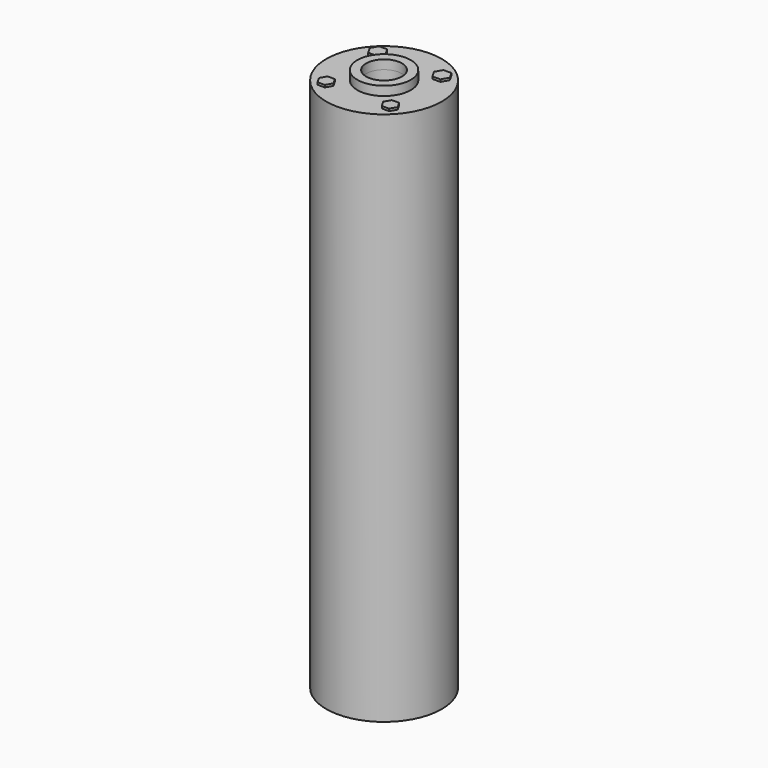
from build123d import *

# Parameters (mm, degrees)
F0_R      = 12.954
F0_R_2    = 5.9944
F0_R_3    = 4.0132
F1_DEPTH  = 119.888
F2_R      = 5.9944
F2_R_2    = 4.0132
F3_DEPTH  = 2.032
F5_R      = 5.9944
F5_R_2    = 4.0132
F6_DEPTH  = 2.032
F7_R      = 4.0132
F8_DEPTH  = 50.8
F10_DEPTH = 0.508


# Not quite as in the source:
# - the program builds the solid bodies; features that only make, move or delete a surface that nothing else refers to are left out


with BuildPart() as f1:
    # F0 (on Top) → F1 (new body)
    with BuildSketch(Plane.XY):
        Circle(F0_R)
        Circle(F0_R_2, mode=Mode.SUBTRACT)
        Circle(F0_R_2)
        Circle(F0_R_3, mode=Mode.SUBTRACT)
        Circle(F0_R_3)
    extrude(amount=F1_DEPTH)

    # F2 (on face) → F3 (join)
    with BuildSketch(Plane.XY.offset(119.888)):
        Circle(F2_R)
        Circle(F2_R_2, mode=Mode.SUBTRACT)
    extrude(amount=F3_DEPTH)

    # F5 (on face) + F0 (on Top) → F6 (join)
    with BuildSketch(Plane.XY):
        Circle(F5_R)
        Circle(F5_R_2, mode=Mode.SUBTRACT)
    with BuildSketch(Plane.XY):
        Circle(F0_R_2)
        Circle(F0_R_3, mode=Mode.SUBTRACT)
    extrude(amount=-F6_DEPTH)

    # F7 (on face) → F8 (cut)
    with BuildSketch(Plane.XY.offset(121.92)):
        Circle(F7_R)
    extrude(amount=-F8_DEPTH, mode=Mode.SUBTRACT)

    # F9 (on face) → F10 (join)
    with BuildSketch(Plane.XY.offset(119.888)):
        Polygon((5.5737421783, -7.205022499), (7.205022499, -7.205022499), (7.205022499, -5.7922923006), (6.3893823387, -5.7922923006), align=None)
        Polygon((7.205022499, -5.7922923006), (7.205022499, -7.205022499), (5.5737421783, -7.205022499), (6.3893823387, -8.6177526973), (8.0206626593, -8.6177526973), (8.8363028196, -7.205022499), (8.0206626593, -5.7922923006), align=None)
        Polygon((-6.3893823387, -8.6177526973), (-5.5737421783, -7.205022499), (-7.205022499, -7.205022499), (-7.205022499, -5.7922923006), (-8.0206626593, -5.7922923006), (-8.8363028196, -7.205022499), (-8.0206626593, -8.6177526973), align=None)
        Polygon((-7.205022499, -7.205022499), (-5.5737421783, -7.205022499), (-6.3893823387, -5.7922923006), (-7.205022499, -5.7922923006), align=None)
        Polygon((-7.205022499, 7.205022499), (-7.205022499, 5.6622778066), (-6.3143184355, 5.6622778066), (-5.4236143721, 7.205022499), align=None)
        Polygon((-8.0957265624, 5.6622778066), (-7.205022499, 5.6622778066), (-7.205022499, 7.205022499), (-5.4236143721, 7.205022499), (-6.3143184355, 8.7477671914), (-8.0957265624, 8.7477671914), (-8.9864306259, 7.205022499), align=None)
        Polygon((7.205022499, 7.205022499), (7.205022499, 5.6622778066), (8.0957265624, 5.6622778066), (8.9864306259, 7.205022499), (8.0957265624, 8.7477671914), (6.3143184355, 8.7477671914), (5.4236143721, 7.205022499), align=None)
        Polygon((6.3143184355, 5.6622778066), (7.205022499, 5.6622778066), (7.205022499, 7.205022499), (5.4236143721, 7.205022499), align=None)
    extrude(amount=F10_DEPTH)


solid = f1.part
